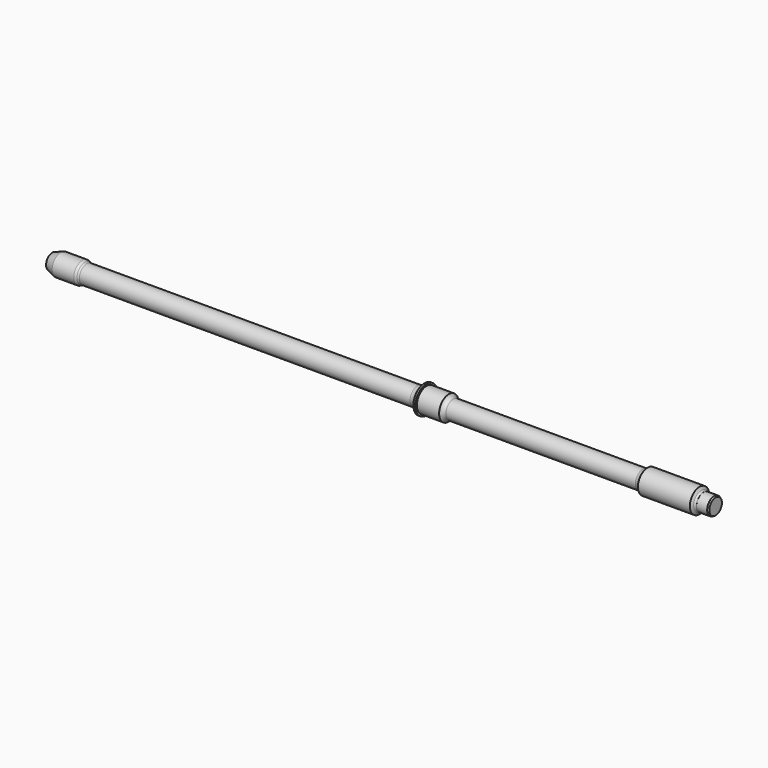
from build123d import *

# Parameters (mm, degrees)
F4_R = 0.25
F5_R = 5
F6_R = 5


# Not quite as in the source:
# - a fillet or chamfer that OpenCascade refuses, or shapes differently, is made with other operations: its cross-section is extruded or revolved along the edge and cut away or added


with BuildPart() as f1:
    # F0 (on Front) → F1 (revolve)
    with BuildSketch(Plane.XZ):
        with BuildLine():
            Line((-2, 9.525), (-350.6009565311, 9.525))
            Line((-350.6009565311, 9.525), (-354, 11.11))
            Line((-354, 11.11), (-376.25, 11.11))
            Line((-376.25, 11.11), (-385, 8))
            Line((-385, 8), (-385, 0))
            Line((-385, 0), (297.49, 0))
            Line((297.49, 0), (297.49, 8.1239745962))
            Line((297.49, 8.1239745962), (295.99, 8.99))
            Line((295.99, 8.99), (285.0470138467, 8.99))
            ThreePointArc((285.0470138467, 8.99), (283.6876657265, 8.797737003), (282.5958183581, 9.63))
            Line((282.5958183581, 9.63), (280.97, 12.446))
            Line((280.97, 12.446), (227.5, 12.446))
            Line((227.5, 12.446), (224.579, 9.525))
            Line((224.579, 9.525), (23, 9.525))
            Line((23, 9.525), (23, 12.495))
            Line((23, 12.495), (0, 12.495))
            Line((0, 12.495), (0, 14.35))
            Line((0, 14.35), (-2, 14.35))
            Line((-2, 14.35), (-2, 9.525))
        make_face()
    revolve(axis=Axis((-43.755, 0, 0), (-1, 0, 0)))

    # F2: fillet of radius 8 on 1 edges, made by hand

    # F2_s1 → F2_t2 (revolve)
    with BuildSketch(Plane.XZ):
        with BuildLine():
            ThreePointArc((-2, 14.35), (-4.9498048155, 10.8391941398), (-9.3429813428, 9.525))
            Line((-9.3429813428, 9.525), (-2, 9.525))
            Line((-2, 9.525), (-2, 14.35))
        make_face()
    revolve(axis=Axis((-2, 0, 0), (-1, 0, 0)))

    # F3: fillet of radius 5 on 1 edges, made by hand

    # F3_s1 → F3_t2 (revolve)
    with BuildSketch(Plane.XZ):
        with BuildLine():
            ThreePointArc((27.5693653826, 9.525), (24.8444800639, 10.3327452367), (23, 12.495))
            Line((23, 12.495), (23, 9.525))
            Line((23, 9.525), (27.5693653826, 9.525))
        make_face()
    revolve(axis=Axis((23, 0, 0), (-1, 0, 0)))

    # F4
    f4_edges = [f1.edges().sort_by_distance(p)[0] for p in [
        (0, 0, -12.495),
    ]]
    fillet(f4_edges, radius=F4_R)

    # F5
    f5_edges = [f1.edges().sort_by_distance(p)[0] for p in [
        (-350.600957, 0, -9.525),
    ]]
    fillet(f5_edges, radius=F5_R)

    # F6
    f6_edges = [f1.edges().sort_by_distance(p)[0] for p in [
        (224.579, 0, -9.525),
    ]]
    fillet(f6_edges, radius=F6_R)


solid = f1.part
